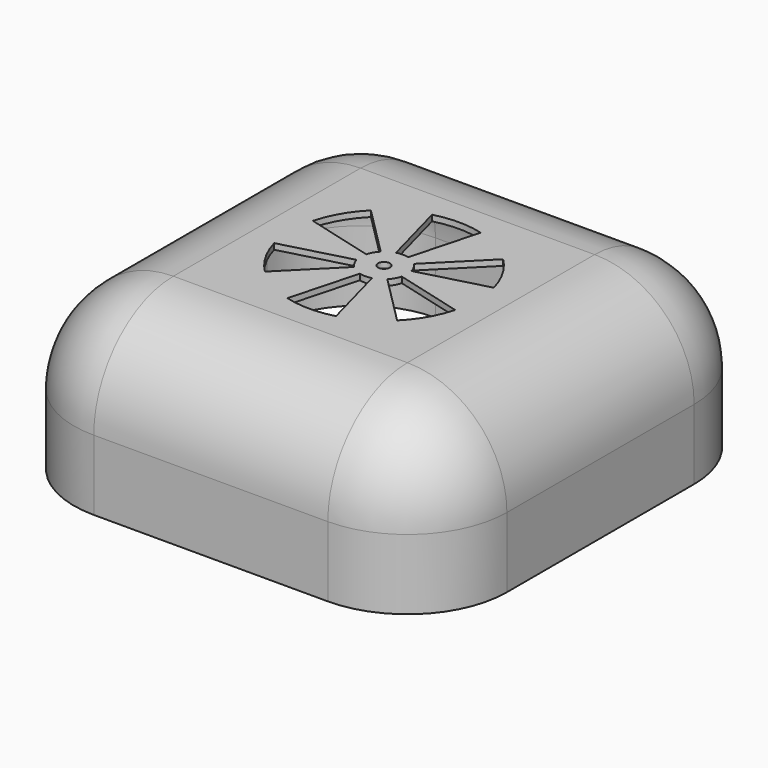
from build123d import *

# Parameters (mm, degrees)
F2_W         = 180
F2_H         = 180
F3_W         = 180
F3_H         = 180
F5_R         = 40
F6_T1_DEPTH  = 130
F6_S5_W      = 40
F6_S5_H      = 40
F6_T6_DEPTH  = 40
F6_S11_W     = 40
F6_S11_H     = 40
F6_T12_DEPTH = 40
F6_S17_W     = 40
F6_S17_H     = 40
F6_T18_DEPTH = 40
F6_S23_W     = 40
F6_S23_H     = 40
F6_T24_DEPTH = 40
F7_T         = 2.5
F0_R         = 2.5
F8_DEPTH     = 2.501


# Not quite as in the source:
# - a fillet or chamfer that OpenCascade refuses, or shapes differently, is made with other operations: its cross-section is extruded or revolved along the edge and cut away or added


with BuildPart() as f4:
    # F2 (on offset) → F4 section 0
    with BuildSketch(Plane.XY.offset(-70)):
        Rectangle(F2_W, F2_H)
    # F3 (on Top) → F4 section 1
    with BuildSketch(Plane.XY):
        Rectangle(F3_W, F3_H)
    loft()

    # F5
    f5_edges = [f4.edges().sort_by_distance(p)[0] for p in [
        (90, 0, 0),
        (0, -90, 0),
        (-90, 0, 0),
        (0, 90, 0),
    ]]
    fillet(f5_edges, radius=F5_R)

    # F6: fillet of radius 40 on 4 edges, made by hand

    # F6_s2 → F6_t1 (cut)
    with BuildSketch(Plane.XY.offset(-170)):
        with BuildLine():
            ThreePointArc((90, -50), (78.2842712475, -78.2842712475), (50, -90))
            Line((50, -90), (90, -90))
            Line((90, -90), (90, -50))
        make_face()
        with BuildLine():
            ThreePointArc((50, 90), (78.2842712475, 78.2842712475), (90, 50))
            Line((90, 50), (90, 90))
            Line((90, 90), (50, 90))
        make_face()
        with BuildLine():
            ThreePointArc((-50, 90), (-78.2842712475, 78.2842712475), (-90, 50))
            Line((-90, 50), (-90, 90))
            Line((-90, 90), (-50, 90))
        make_face()
        with BuildLine():
            ThreePointArc((-90, -50), (-78.2842712475, -78.2842712475), (-50, -90))
            Line((-50, -90), (-90, -90))
            Line((-90, -90), (-90, -50))
        make_face()
    extrude(amount=F6_T1_DEPTH, mode=Mode.SUBTRACT)


with BuildPart() as f6_tool4:
    # F6_s5 → F6_t6 (new body)
    with BuildSketch(Plane.YZ.offset(-50)):
        with Locations((-70, -20)):
            Rectangle(F6_S5_W, F6_S5_H)
    extrude(amount=-F6_T6_DEPTH)

    # F6_s7 → F6_t8 (revolve, cut)
    with BuildSketch(Plane(origin=(-50, -50, -40), x_dir=(0, 0.7071067812, -0.7071067812), z_dir=(0, 0.7071067812, 0.7071067812))):
        with BuildLine():
            ThreePointArc((0, -40), (40, 0), (0, 40))
            Line((0, 40), (0, -40))
        make_face()
    revolve(axis=Axis((-50, -50, -40), (-1, 0, 0)), mode=Mode.SUBTRACT)


with BuildPart() as f4_1:
    add(f4.part)

    # F6_t3: cut F6_tool4
    add(f6_tool4.part, mode=Mode.SUBTRACT)


with BuildPart() as f6_tool10:
    # F6_s11 → F6_t12 (new body)
    with BuildSketch(Plane.XZ.offset(-50)):
        with Locations((-70, -20)):
            Rectangle(F6_S11_W, F6_S11_H)
    extrude(amount=-F6_T12_DEPTH)

    # F6_s13 → F6_t14 (revolve, cut)
    with BuildSketch(Plane(origin=(-50, 50, -40), x_dir=(0.7071067812, 0, -0.7071067812), z_dir=(0.7071067812, 0, 0.7071067812))):
        with BuildLine():
            ThreePointArc((0, -40), (40, 0), (0, 40))
            Line((0, 40), (0, -40))
        make_face()
    revolve(axis=Axis((-50, 50, -40), (0, 1, 0)), mode=Mode.SUBTRACT)


with BuildPart() as f4_2:
    add(f4_1.part)

    # F6_t9: cut F6_tool10
    add(f6_tool10.part, mode=Mode.SUBTRACT)


with BuildPart() as f6_tool16:
    # F6_s17 → F6_t18 (new body)
    with BuildSketch(Plane.XZ.offset(-50)):
        with Locations((70, -20)):
            Rectangle(F6_S17_W, F6_S17_H)
    extrude(amount=-F6_T18_DEPTH)

    # F6_s19 → F6_t20 (revolve, cut)
    with BuildSketch(Plane(origin=(50, 50, -40), x_dir=(-0.7071067812, 0, -0.7071067812), z_dir=(0.7071067812, 0, -0.7071067812))):
        with BuildLine():
            ThreePointArc((0, -40), (40, 0), (0, 40))
            Line((0, 40), (0, -40))
        make_face()
    revolve(axis=Axis((50, 50, -40), (0, 1, 0)), mode=Mode.SUBTRACT)


with BuildPart() as f4_3:
    add(f4_2.part)

    # F6_t15: cut F6_tool16
    add(f6_tool16.part, mode=Mode.SUBTRACT)


with BuildPart() as f6_tool22:
    # F6_s23 → F6_t24 (new body)
    with BuildSketch(Plane.YZ.offset(50)):
        with Locations((-70, -20)):
            Rectangle(F6_S23_W, F6_S23_H)
    extrude(amount=F6_T24_DEPTH)

    # F6_s25 → F6_t26 (revolve, cut)
    with BuildSketch(Plane(origin=(50, -50, -40), x_dir=(0, 0.7071067812, -0.7071067812), z_dir=(0, -0.7071067812, -0.7071067812))):
        with BuildLine():
            ThreePointArc((0, -40), (40, 0), (0, 40))
            Line((0, 40), (0, -40))
        make_face()
    revolve(axis=Axis((50, -50, -40), (1, 0, 0)), mode=Mode.SUBTRACT)


with BuildPart() as f4_4:
    add(f4_3.part)

    # F6_t21: cut F6_tool22
    add(f6_tool22.part, mode=Mode.SUBTRACT)

    # F7
    f7_openings = [f4_4.faces().sort_by_distance(p)[0] for p in [
        (0, 0, -70),
    ]]
    offset(amount=F7_T, openings=f7_openings)

    # F0 (on Top) → F8 (cut, through all)
    with BuildSketch(Plane.XY):
        with BuildLine():
            Line((-10.4, 38.6243446546), (-2.6, 9.6560861637))
            ThreePointArc((-2.6, 9.6560861637), (0, 10), (2.6, 9.6560861637))
            Line((2.6, 9.6560861637), (10.4, 38.6243446546))
            ThreePointArc((10.4, 38.6243446546), (0, 40), (-10.4, 38.6243446546))
        make_face()
        with BuildLine():
            ThreePointArc((-9.6624159189, 2.576377032), (-8.6602540378, 5), (-7.0624159189, 7.0797091317))
            Line((-7.0624159189, 7.0797091317), (-28.2496636754, 28.3188365267))
            ThreePointArc((-28.2496636754, 28.3188365267), (-34.6410161514, 20), (-38.6496636754, 10.305508128))
            Line((-38.6496636754, 10.305508128), (-9.6624159189, 2.576377032))
        make_face()
        with BuildLine():
            ThreePointArc((-7.0624159189, -7.0797091317), (-8.6602540378, -5), (-9.6624159189, -2.576377032))
            Line((-9.6624159189, -2.576377032), (-38.6496636754, -10.305508128))
            ThreePointArc((-38.6496636754, -10.305508128), (-34.6410161514, -20), (-28.2496636754, -28.3188365267))
            Line((-28.2496636754, -28.3188365267), (-7.0624159189, -7.0797091317))
        make_face()
        with BuildLine():
            ThreePointArc((2.6, -9.6560861637), (0, -10), (-2.6, -9.6560861637))
            Line((-2.6, -9.6560861637), (-10.4, -38.6243446546))
            ThreePointArc((-10.4, -38.6243446546), (0, -40), (10.4, -38.6243446546))
            Line((10.4, -38.6243446546), (2.6, -9.6560861637))
        make_face()
        with BuildLine():
            ThreePointArc((9.6624159189, -2.576377032), (8.6602540378, -5), (7.0624159189, -7.0797091317))
            Line((7.0624159189, -7.0797091317), (28.2496636754, -28.3188365267))
            ThreePointArc((28.2496636754, -28.3188365267), (34.6410161514, -20), (38.6496636754, -10.305508128))
            Line((38.6496636754, -10.305508128), (9.6624159189, -2.576377032))
        make_face()
        with BuildLine():
            ThreePointArc((7.0624159189, 7.0797091317), (8.6602540378, 5), (9.6624159189, 2.576377032))
            Line((9.6624159189, 2.576377032), (38.6496636754, 10.305508128))
            ThreePointArc((38.6496636754, 10.305508128), (34.6410161514, 20), (28.2496636754, 28.3188365267))
            Line((28.2496636754, 28.3188365267), (7.0624159189, 7.0797091317))
        make_face()
        Circle(F0_R)
    extrude(amount=F8_DEPTH, mode=Mode.SUBTRACT)


solid = f4_4.part
